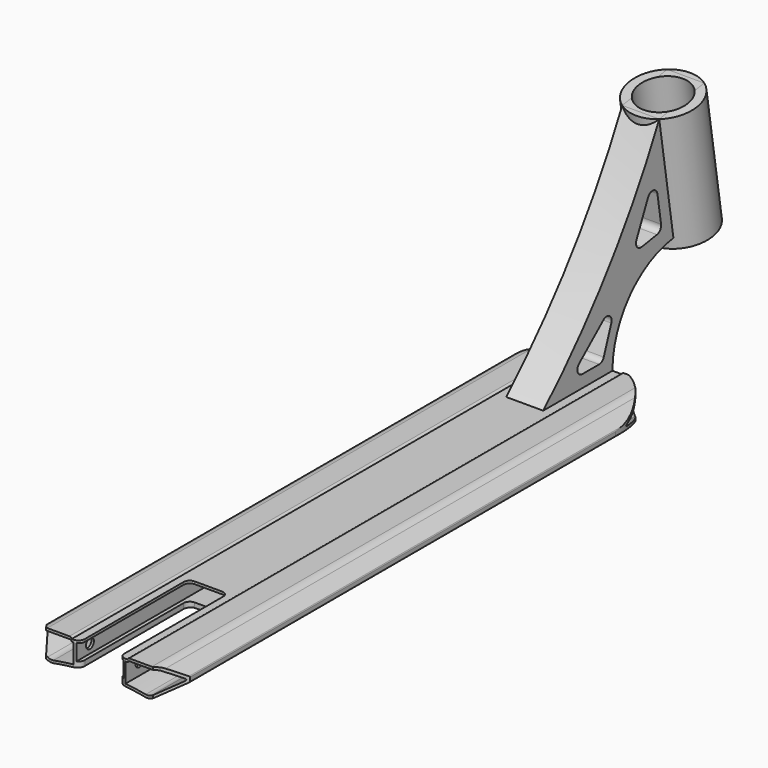
from build123d import *

# Parameters (mm, degrees)
F1_DEPTH       = 250
F2_W           = 38
F2_H           = 13
F3_DEPTH       = 250
F5_T1_DEPTH    = 509.3674969976
F6_R           = 9
F7_R           = 1
F8_DEPTH       = 500.001
F10_DEPTH      = 22.2193051812
F10_DEPTH_BACK = 1.301
F12_DEPTH      = 22.219305294
F12_DEPTH_BACK = 1.3010001
F13_T1_DEPTH   = 2
F13_T6_DEPTH   = 32
F13_S7_R       = 200
F13_T8_DEPTH   = 18
F13_T13_DEPTH  = 64.2634824315
F13_T19_DEPTH  = 34.2634824315
F13_S20_R      = 200
F13_T21_DEPTH  = 19
F13_T25_DEPTH  = 34.2634824315
F13_S26_R      = 200
F13_T27_DEPTH  = 19
F13_T31_DEPTH  = 64.2634824315
F13_T37_DEPTH  = 32
F13_S38_R      = 200
F13_T39_DEPTH  = 18
F13_T41_DEPTH  = 64.2634824315
F13_T43_DEPTH  = 62
F15_DEPTH      = 15
F16_R          = 27.5
F17_DEPTH      = 100
F19_D          = 40
F21_D          = 8
F21_DEPTH      = 50
F21_TIP        = 2.4034424761
F23_DEPTH      = 72.5010001
F24_R          = 5


# Not quite as in the source:
# - a fillet or chamfer that OpenCascade refuses, or shapes differently, is made with other operations: its cross-section is extruded or revolved along the edge and cut away or added


with BuildPart() as f1:
    # F0 (on Front) → F1 (new body, symmetric)
    with BuildSketch(Plane.XZ):
        with BuildLine():
            Line((22.5, 0), (0, 0))
            Line((0, 0), (-22.5, 0))
            Line((-22.5, 0), (-22.5, 1.3))
            Line((-22.5, 1.3), (-45.5824640741, 1.3))
            Line((-45.5824640741, 1.3), (-57.5, -8.7))
            Line((-57.5, -8.7), (-57.5, -12.7))
            Line((-57.5, -12.7), (-40.1794919243, -22.7))
            ThreePointArc((-40.1794919243, -22.7), (0, -18.6224551416), (40.1794919243, -22.7))
            Line((40.1794919243, -22.7), (57.5, -12.7))
            Line((57.5, -12.7), (57.5, -8.7))
            Line((57.5, -8.7), (45.5824640741, 1.3))
            Line((45.5824640741, 1.3), (22.5, 1.3))
            Line((22.5, 1.3), (22.5, 0))
        make_face()
    extrude(amount=F1_DEPTH, both=True)

    # F2 (on Front) → F3 (cut, symmetric)
    with BuildSketch(Plane.XZ):
        with Locations((0, -8.5)):
            Rectangle(F2_W, F2_H)
    extrude(amount=F3_DEPTH, both=True, mode=Mode.SUBTRACT)

    # F5: fillet of radius 2 on 2 edges, made by hand

    # F5_s2 → F5_t1 (cut)
    with BuildSketch(Plane.XZ.offset(-254.6837484988)):
        with BuildLine():
            ThreePointArc((-24.3734993995, 1.3), (-23.2333239744, 0.9431676725), (-22.5, 0))
            Line((-22.5, 0), (-22.5, 1.3))
            Line((-22.5, 1.3), (-24.3734993995, 1.3))
        make_face()
        with BuildLine():
            ThreePointArc((24.3734993995, 1.3), (23.2333239744, 0.9431676725), (22.5, 0))
            Line((22.5, 0), (22.5, 1.3))
            Line((22.5, 1.3), (24.3734993995, 1.3))
        make_face()
    extrude(amount=F5_T1_DEPTH, mode=Mode.SUBTRACT)

    # F6
    f6_edges = [f1.edges().sort_by_distance(p)[0] for p in [
        (-40.179492, 0, -22.7),
        (-45.582464, 0, 1.3),
        (40.179492, 0, -22.7),
        (45.582464, 0, 1.3),
    ]]
    fillet(f6_edges, radius=F6_R)

    # F7
    f7_edges = [f1.edges().sort_by_distance(p)[0] for p in [
        (-57.5, 0, -8.7),
        (-57.5, 0, -12.7),
        (57.5, 0, -8.7),
        (57.5, 0, -12.7),
    ]]
    fillet(f7_edges, radius=F7_R)

    # F4 (on face) → F8 (cut, through all)
    with BuildSketch(Plane.XZ.offset(250)):
        with BuildLine():
            Line((22.5, -2), (21, -2))
            Line((21, -2), (21, -17.7170047426))
            ThreePointArc((21, -17.7170047426), (29.1789785809, -18.7410222645), (37.3093701274, -20.0978700124))
            ThreePointArc((37.3093701274, -20.0978700124), (39.7790673433, -20.1186780608), (42.1022690923, -19.2804830077))
            Line((42.1022690923, -19.2804830077), (55.6135241478, -11.4797562644))
            ThreePointArc((55.6135241478, -11.4797562644), (56.1097188459, -10.7008866033), (55.7563117574, -9.8476864174))
            Line((55.7563117574, -9.8476864174), (46.8062452335, -2.3376888982))
            ThreePointArc((46.8062452335, -2.3376888982), (44.7008729689, -1.1221516545), (42.3067319657, -0.7))
            Line((42.3067319657, -0.7), (24.3734993995, -0.7))
            ThreePointArc((24.3734993995, -0.7), (23.2333239744, -1.0568323275), (22.5, -2))
        make_face()
        with BuildLine():
            ThreePointArc((-22.5, -2), (-23.2333239744, -1.0568323275), (-24.3734993995, -0.7))
            Line((-24.3734993995, -0.7), (-42.3067319657, -0.7))
            ThreePointArc((-42.3067319657, -0.7), (-44.7008729689, -1.1221516545), (-46.8062452335, -2.3376888982))
            Line((-46.8062452335, -2.3376888982), (-55.7563117574, -9.8476864174))
            ThreePointArc((-55.7563117574, -9.8476864174), (-56.1097188459, -10.7008866033), (-55.6135241478, -11.4797562644))
            Line((-55.6135241478, -11.4797562644), (-42.1022690923, -19.2804830077))
            ThreePointArc((-42.1022690923, -19.2804830077), (-39.7790673433, -20.1186780608), (-37.3093701274, -20.0978700124))
            ThreePointArc((-37.3093701274, -20.0978700124), (-29.1789785809, -18.7410222645), (-21, -17.7170047426))
            Line((-21, -17.7170047426), (-21, -2))
            Line((-21, -2), (-22.5, -2))
        make_face()
    extrude(amount=-F8_DEPTH, mode=Mode.SUBTRACT)

    # F9 (on Top) → F10 (cut, two sides)
    with BuildSketch(Plane.XY) as f10_sk:
        with BuildLine():
            ThreePointArc((-57.5, 200), (0, 257.5), (57.5, 200))
            Line((57.5, 200), (57.5, 280))
            Line((57.5, 280), (-57.5, 280))
            Line((-57.5, 280), (-57.5, 200))
        make_face()
    extrude(amount=-F10_DEPTH, mode=Mode.SUBTRACT)
    extrude(f10_sk.sketch, amount=F10_DEPTH_BACK, mode=Mode.SUBTRACT)

    # F11 (on Top) → F12 (cut, two sides)
    with BuildSketch(Plane.XY) as f12_sk:
        Polygon((-43.2975540478, -250), (-68, -216), (-68, -346), (68, -346), (68, -216), (43.2975540478, -250), (16, -250), (16, -140), (-16, -140), (-16, -250), align=None)
    extrude(amount=-F12_DEPTH, mode=Mode.SUBTRACT)
    extrude(f12_sk.sketch, amount=F12_DEPTH_BACK, mode=Mode.SUBTRACT)

    # F13: fillet of radius 5 on 7 edges, made by hand

    # F13_s2 → F13_t1 (join)
    with BuildSketch(Plane.XY.offset(-2)):
        with BuildLine():
            ThreePointArc((-11, -140), (-14.5355339059, -141.4644660941), (-16, -145))
            Line((-16, -145), (-16.1, -145))
            Line((-16.1, -145), (-16.1, -139.9))
            Line((-16.1, -139.9), (-11, -139.9))
            Line((-11, -139.9), (-11, -140))
        make_face()
        with BuildLine():
            ThreePointArc((16, -145), (14.5355339059, -141.4644660941), (11, -140))
            Line((11, -140), (11, -139.9))
            Line((11, -139.9), (16.1, -139.9))
            Line((16.1, -139.9), (16.1, -145))
            Line((16.1, -145), (16, -145))
        make_face()
    extrude(amount=F13_T1_DEPTH)


with BuildPart() as f13_tool4:
    # F13_s5 → F13_t6 (new body)
    with BuildSketch(Plane.XY):
        with BuildLine():
            ThreePointArc((-11, -140), (-14.5355339059, -141.4644660941), (-16, -145))
            Line((-16, -145), (-16.1, -145))
            Line((-16.1, -145), (-16.1, -139.9))
            Line((-16.1, -139.9), (-11, -139.9))
            Line((-11, -139.9), (-11, -140))
        make_face()
    extrude(amount=-F13_T6_DEPTH)

    # F13_s7 → F13_t8 (cut, symmetric)
    with BuildSketch(Plane.XZ.offset(142.4)):
        with Locations((0, -218.6224551416)):
            Circle(F13_S7_R)
    extrude(amount=F13_T8_DEPTH, both=True, mode=Mode.SUBTRACT)

    split(bisect_by=Plane.XY.offset(-15), keep=Keep.BOTTOM)


with BuildPart() as f1_1:
    add(f1.part)

    # F13_t3: union F13_tool4
    add(f13_tool4.part)


with BuildPart() as f13_tool11:
    # F13_s12 → F13_t13 (new body)
    with BuildSketch(Plane.XY.offset(15)):
        with BuildLine():
            ThreePointArc((-16, -145), (-14.5355339059, -141.4644660941), (-11, -140))
            Line((-11, -140), (-11, -139.9))
            Line((-11, -139.9), (-16.1, -139.9))
            Line((-16.1, -139.9), (-16.1, -145))
            Line((-16.1, -145), (-16, -145))
        make_face()
    extrude(amount=-F13_T13_DEPTH)

    split(bisect_by=Plane.XY.offset(-2), keep=Keep.TOP)

    split(bisect_by=Plane.XY, keep=Keep.BOTTOM)


with BuildPart() as f1_2:
    add(f1_1.part)

    # F13_t10: union F13_tool11
    add(f13_tool11.part)


with BuildPart() as f13_tool17:
    # F13_s18 → F13_t19 (new body)
    with BuildSketch(Plane.XY.offset(-15)):
        with BuildLine():
            ThreePointArc((-16, -145), (-14.5355339059, -141.4644660941), (-11, -140))
            Line((-11, -140), (-11, -139.9))
            Line((-11, -139.9), (-16.1, -139.9))
            Line((-16.1, -139.9), (-16.1, -145))
            Line((-16.1, -145), (-16, -145))
        make_face()
    extrude(amount=-F13_T19_DEPTH)

    # F13_s20 → F13_t21 (cut, symmetric)
    with BuildSketch(Plane.XZ.offset(142.4)):
        with Locations((0, -218.6224551416)):
            Circle(F13_S20_R)
    extrude(amount=F13_T21_DEPTH, both=True, mode=Mode.SUBTRACT)


with BuildPart() as f1_3:
    add(f1_2.part)

    # F13_t16: union F13_tool17
    add(f13_tool17.part)


with BuildPart() as f13_tool23:
    # F13_s24 → F13_t25 (new body)
    with BuildSketch(Plane.XY.offset(-49.2634824315)):
        with BuildLine():
            ThreePointArc((16, -145), (14.5355339059, -141.4644660941), (11, -140))
            Line((11, -140), (11, -139.9))
            Line((11, -139.9), (16.1, -139.9))
            Line((16.1, -139.9), (16.1, -145))
            Line((16.1, -145), (16, -145))
        make_face()
    extrude(amount=F13_T25_DEPTH)

    # F13_s26 → F13_t27 (cut, symmetric)
    with BuildSketch(Plane.XZ.offset(142.4)):
        with Locations((0, -218.6224551416)):
            Circle(F13_S26_R)
    extrude(amount=F13_T27_DEPTH, both=True, mode=Mode.SUBTRACT)


with BuildPart() as f1_4:
    add(f1_3.part)

    # F13_t22: union F13_tool23
    add(f13_tool23.part)


with BuildPart() as f13_tool29:
    # F13_s30 → F13_t31 (new body)
    with BuildSketch(Plane.XY.offset(-49.2634824315)):
        with BuildLine():
            ThreePointArc((16, -145), (14.5355339059, -141.4644660941), (11, -140))
            Line((11, -140), (11, -139.9))
            Line((11, -139.9), (16.1, -139.9))
            Line((16.1, -139.9), (16.1, -145))
            Line((16.1, -145), (16, -145))
        make_face()
    extrude(amount=F13_T31_DEPTH)

    split(bisect_by=Plane.XY.offset(-2), keep=Keep.TOP)

    split(bisect_by=Plane.XY, keep=Keep.BOTTOM)


with BuildPart() as f1_5:
    add(f1_4.part)

    # F13_t28: union F13_tool29
    add(f13_tool29.part)


with BuildPart() as f13_tool35:
    # F13_s36 → F13_t37 (new body)
    with BuildSketch(Plane.XY.offset(-32)):
        with BuildLine():
            ThreePointArc((16, -145), (14.5355339059, -141.4644660941), (11, -140))
            Line((11, -140), (11, -139.9))
            Line((11, -139.9), (16.1, -139.9))
            Line((16.1, -139.9), (16.1, -145))
            Line((16.1, -145), (16, -145))
        make_face()
    extrude(amount=F13_T37_DEPTH)

    # F13_s38 → F13_t39 (cut, symmetric)
    with BuildSketch(Plane.XZ.offset(142.4)):
        with Locations((0, -218.6224551416)):
            Circle(F13_S38_R)
    extrude(amount=F13_T39_DEPTH, both=True, mode=Mode.SUBTRACT)

    split(bisect_by=Plane.XY.offset(-15), keep=Keep.BOTTOM)


with BuildPart() as f1_6:
    add(f1_5.part)

    # F13_t34: union F13_tool35
    add(f13_tool35.part)

    # F13_s42 → F13_t41 (cut)
    with BuildSketch(Plane.XY.offset(-49.2634824315)):
        with BuildLine():
            ThreePointArc((-21, -250), (-17.4644660941, -248.5355339059), (-16, -245))
            Line((-16, -245), (-15.9, -245))
            Line((-15.9, -245), (-15.9, -250.1))
            Line((-15.9, -250.1), (-21, -250.1))
            Line((-21, -250.1), (-21, -250))
        make_face()
        with BuildLine():
            ThreePointArc((21, -250), (17.4644660941, -248.5355339059), (16, -245))
            Line((16, -245), (15.9, -245))
            Line((15.9, -245), (15.9, -250.1))
            Line((15.9, -250.1), (21, -250.1))
            Line((21, -250.1), (21, -250))
        make_face()
    extrude(amount=F13_T41_DEPTH, mode=Mode.SUBTRACT)

    # F13_s44 → F13_t43 (cut)
    with BuildSketch(Plane.XY.offset(-32)):
        with BuildLine():
            ThreePointArc((21, -250), (17.4644660941, -248.5355339059), (16, -245))
            Line((16, -245), (15.9, -245))
            Line((15.9, -245), (15.9, -250.1))
            Line((15.9, -250.1), (21, -250.1))
            Line((21, -250.1), (21, -250))
        make_face()
    extrude(amount=F13_T43_DEPTH, mode=Mode.SUBTRACT)

    # F14 (on Right) → F15 (join, symmetric)
    with BuildSketch(Plane.YZ):
        with BuildLine():
            ThreePointArc((297.3819995028, 160), (245.9666940414, 74.662277853), (180, 0))
            Line((180, 0), (250, 0))
            ThreePointArc((250, 0), (267.6550746197, 46.4758946867), (311.7145367693, 69.5079211245))
            Line((311.7145367693, 69.5079211245), (313.0254460068, 61.2311659405))
            Line((313.0254460068, 61.2311659405), (358.4591096742, 68.4271513323))
            Line((358.4591096742, 68.4271513323), (342.8156631702, 167.1959853919))
            Line((342.8156631702, 167.1959853919), (297.3819995028, 160))
        make_face()
    extrude(amount=F15_DEPTH, both=True)

    # F16 (on face) → F17 (join, through all)
    with BuildSketch(Plane(origin=(0, -17.4439040266, 110.1364754698), x_dir=(1, 0, 0), z_dir=(0, -0.156434465, 0.9876883406))):
        with Locations((0, 341.7502480182)):
            Circle(F16_R)
    extrude(amount=-F17_DEPTH)

    # F19 (through all)
    with Locations(Plane(origin=(0, -17.4439040266, 110.1364754698), x_dir=(1, 0, 0), z_dir=(0, -0.156434465, 0.9876883406))):
        with Locations((0, 341.7502480182)):
            Hole(F19_D / 2)

    # F21 (one way)
    with BuildSketch(Plane.YZ.offset(21)):
        with Locations((-236, -7.7170047426)):
            Circle(F21_D / 2)
    extrude(amount=-F21_DEPTH, mode=Mode.SUBTRACT)
    with Locations(Plane.YZ.offset(21)):
        with Locations((-236, -7.7170047426)):
            with Locations((0, 0, -(F21_DEPTH + F21_TIP / 2))):  # 118° drill point
                Cone(0, F21_D / 2, F21_TIP, mode=Mode.SUBTRACT)

    # F22 (on face) → F23 (cut, through all)
    with BuildSketch(Plane.YZ.offset(15)):
        Polygon((240, 10), (255.3909064497, 52.2861679354), (206, 10), align=None)
        Polygon((292.9320627918, 123.858919862), (270.3409635007, 74.719910584), (299.9716137186, 79.4129445352), align=None)
    extrude(amount=-F23_DEPTH, mode=Mode.SUBTRACT)

    # F24
    f24_edges = [f1_6.edges().sort_by_distance(p)[0] for p in [
        (0, 240, 10),
        (0, 206, 10),
        (0, 255.390906, 52.286168),
        (0, 292.932063, 123.85892),
        (0, 299.971614, 79.412945),
        (0, 270.340964, 74.719911),
    ]]
    fillet(f24_edges, radius=F24_R)


solid = f1_6.part
